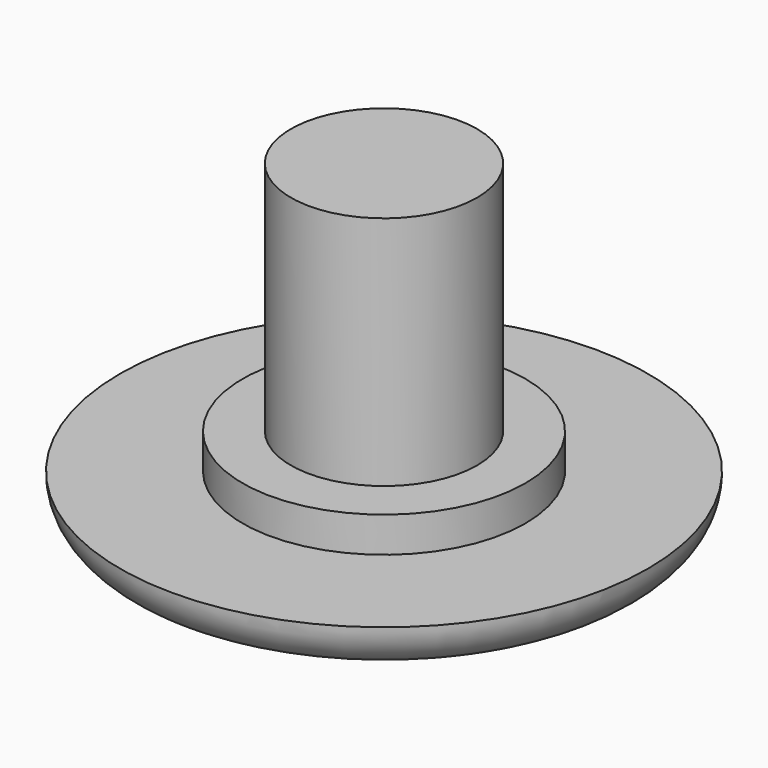
from build123d import *

# Parameters (mm, degrees)
F0_R     = 11.2
F1_DEPTH = 2
F2_R     = 6
F3_DEPTH = 1.5
F4_R     = 3.95
F5_DEPTH = 10
F6_R     = 1.99999


# Not quite as in the source:
# - a fillet or chamfer is up to 0.001 mm smaller than in the source, because OpenCascade refuses the exact size


with BuildPart() as f1:
    # F0 (on Top) → F1 (new body)
    with BuildSketch(Plane.XY):
        Circle(F0_R)
    extrude(amount=F1_DEPTH)

    # F2 (on face) → F3 (join)
    with BuildSketch(Plane.XY.offset(2)):
        Circle(F2_R)
    extrude(amount=F3_DEPTH)

    # F4 (on face) → F5 (join)
    with BuildSketch(Plane.XY.offset(3.5)):
        Circle(F4_R)
    extrude(amount=F5_DEPTH)

    # F6 (radius 2 in the source; OpenCascade refuses exactly that, so slightly less here)
    f6_edges = [f1.edges().sort_by_distance(p)[0] for p in [
        (-11.2, 0, 0),
    ]]
    fillet(f6_edges, radius=F6_R)


solid = f1.part
